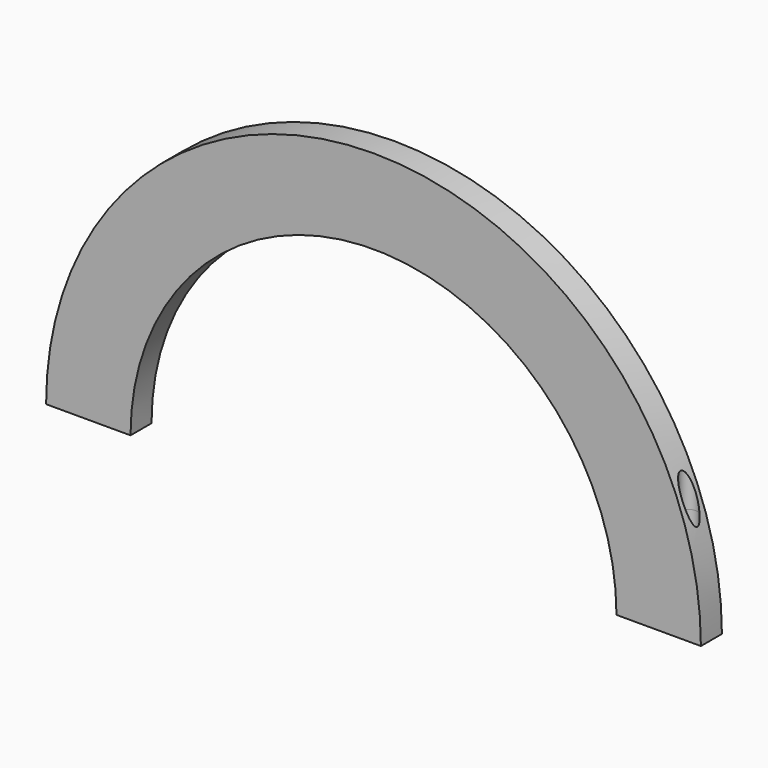
from build123d import *
from build123d import SkipClean  # not in build123d's __all__

# Parameters (mm, degrees)
F1_DEPTH = 7
F2_DEPTH = 6
F4_R     = 4.5
F5_DEPTH = 119.501
F6_DEPTH = 20
F7_R     = 3
F8_DEPTH = 35.0010001


# Not quite as in the source:
# - after a boolean that leaves OpenCascade's solid faulty, fix() repairs it


with BuildPart() as f1:
    # F0 (on Front) → F1 (new body, symmetric)
    with BuildSketch(Plane.XZ):
        with BuildLine():
            Line((129.5, 0), (174.5, 0))
            ThreePointArc((174.5, 0), (0, 174.5), (-174.5, 0))
            Line((-174.5, 0), (-129.5, 0))
            ThreePointArc((-129.5, 0), (0, 129.5), (129.5, 0))
        make_face()
    extrude(amount=F1_DEPTH, both=True)

    # F0 (on Front) → F2 (join, symmetric)
    with BuildSketch(Plane.XZ):
        with BuildLine():
            Line((129.5, 0), (174.5, 0))
            ThreePointArc((174.5, 0), (0, 174.5), (-174.5, 0))
            Line((-174.5, 0), (-129.5, 0))
            ThreePointArc((-129.5, 0), (0, 129.5), (129.5, 0))
        make_face()
    extrude(amount=F2_DEPTH, both=True)

    # F4 (on offset) → F5 (cut, through all)
    with BuildSketch(Plane.XY.offset(55)):
        with Locations((-162.5, 0)):
            Circle(F4_R)
        with Locations((162.5, 0)):
            Circle(F4_R)
    extrude(amount=F5_DEPTH, mode=Mode.SUBTRACT)

    # F4 (on offset) → F6 (cut)
    with BuildSketch(Plane.XY.offset(55)):
        with Locations((-162.5, 0)):
            Circle(F4_R)
        with Locations((162.5, 0)):
            Circle(F4_R)
    with SkipClean():  # cleaning this boolean's faces spoils the solid; the shape is the same uncleaned
        extrude(amount=-F6_DEPTH, mode=Mode.SUBTRACT)

    # F7 (on face) → F8 (cut, through all)
    with BuildSketch(Plane.XY.offset(35)):
        with Locations((-162.5, 0)):
            Circle(F7_R)
        with Locations((162.5, 0)):
            Circle(F7_R)
    extrude(amount=-F8_DEPTH, mode=Mode.SUBTRACT)

    add(f1.part.fix(), mode=Mode.REPLACE)


solid = f1.part
